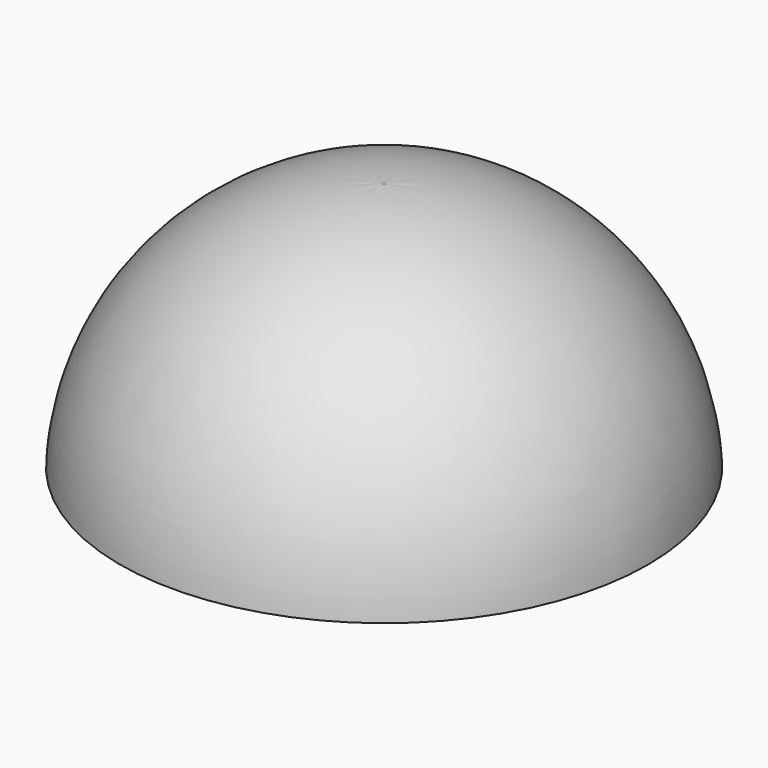
from build123d import *

# Parameters (mm, degrees)
F0_R     = 15.875
F1_DEPTH = 15
F3_R     = 3
F4_DEPTH = 12
F5_R     = 4
F6_DEPTH = 25


# Not quite as in the source:
# - a fillet or chamfer that OpenCascade refuses, or shapes differently, is made with other operations: its cross-section is extruded or revolved along the edge and cut away or added


with BuildPart() as f1:
    # F0 (on Top) → F1 (new body)
    with BuildSketch(Plane.XY):
        Circle(F0_R)
    extrude(amount=F1_DEPTH)

    # F2: fillet of radius 15.8 on 1 edges, made by hand

    # F2_s1 → F2_t2 (revolve, cut)
    with BuildSketch(Plane.XZ):
        with BuildLine():
            ThreePointArc((15.875, 0), (10.9810366905, 10.6516374375), (0.0952661619, 15))
            Line((0.0952661619, 15), (15.875, 15))
            Line((15.875, 15), (15.875, 0))
        make_face()
    revolve(axis=Axis((0, 0, 15), (0, 0, 1)), mode=Mode.SUBTRACT)

    # F3 (on face) → F4 (cut)
    with BuildSketch(Plane(origin=(0, 0, 0), x_dir=(1, 0, 0), z_dir=(0, 0, -1))):
        Circle(F3_R)
    extrude(amount=-F4_DEPTH, mode=Mode.SUBTRACT)

    # F5 (on Right) → F6 (cut)
    with BuildSketch(Plane.YZ):
        Circle(F5_R)
    extrude(amount=-F6_DEPTH, mode=Mode.SUBTRACT)


solid = f1.part
